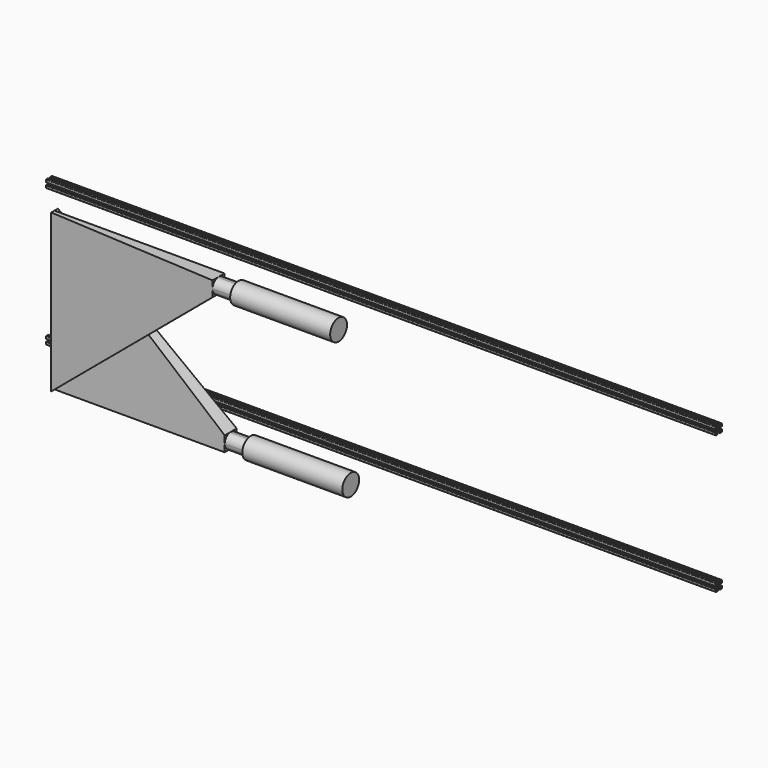
from build123d import *

# Parameters (mm, degrees)
F0_W           = 38.1
F0_H           = 400
F1_DEPTH       = 431.8
F2_SIZE2       = 431.79999
F2_SIZE        = 27.79999
F3_SIZE2       = 27.79999
F3_SIZE        = 431.79999
F4_SIZE2       = 362.19999
F4_SIZE        = 431.79999
F5_SIZE2       = 431.79999
F5_SIZE        = 362.19999
F8_START       = 0.01
F8_DEPTH       = 50.79
F11_START      = 0.01
F9_R           = 26.67
F11_DEPTH      = 253.99
F10_R          = 26.67
F13_DEPTH      = 1600
F13_DEPTH_BACK = 100


# Not quite as in the source:
# - a fillet or chamfer is up to 0.001 mm smaller than in the source, because OpenCascade refuses the exact size
# - ends of sketch curves that miss each other by under 0.0002 mm in the source are joined


with BuildPart() as f1:
    # F0 (on Right) → F1 (new body)
    with BuildSketch(Plane.YZ):
        with Locations((-19.5574148118, 124.7872307897)):
            Rectangle(F0_W, F0_H)
    extrude(amount=F1_DEPTH)

    # F3 (size 431.8 and 27.8 in the source; OpenCascade refuses exactly that, so slightly less here)
    f3_edges = [f1.edges().sort_by_distance(p)[0] for p in [
        (0, -38.607415, 124.787231),
    ]]
    f3_side = f1.faces().sort_by_distance((215.9, -38.607415, 124.787231))[0]
    chamfer(f3_edges, length=F3_SIZE, length2=F3_SIZE2, reference=f3_side)

    # F5 (size 362.2 and 431.8 in the source; OpenCascade refuses exactly that, so slightly less here)
    f5_edges = [f1.edges().sort_by_distance(p)[0] for p in [
        (431.8, -19.557415, -75.212769),
    ]]
    f5_side = f1.faces().sort_by_distance((431.8, -19.557415, 124.787231))[0]
    chamfer(f5_edges, length=F5_SIZE, length2=F5_SIZE2, reference=f5_side)


with BuildPart() as f1b:
    # F0 (on Right) → F1, piece 2 (new body)
    with BuildSketch(Plane.YZ):
        with Locations((19.05, 124.7872307897)):
            Rectangle(F0_W, F0_H)
    extrude(amount=F1_DEPTH)

    # F2 (size 27.8 and 431.8 in the source; OpenCascade refuses exactly that, so slightly less here)
    f2_edges = [f1b.edges().sort_by_distance(p)[0] for p in [
        (0, 38.1, 124.787231),
    ]]
    f2_side = f1b.faces().sort_by_distance((0, 19.05, 124.787231))[0]
    chamfer(f2_edges, length=F2_SIZE, length2=F2_SIZE2, reference=f2_side)

    # F4 (size 431.8 and 362.2 in the source; OpenCascade refuses exactly that, so slightly less here)
    f4_edges = [f1b.edges().sort_by_distance(p)[0] for p in [
        (431.8, 19.05, 324.787231),
    ]]
    f4_side = f1b.faces().sort_by_distance((257.236203, 13.430649, 324.787231))[0]
    chamfer(f4_edges, length=F4_SIZE, length2=F4_SIZE2, reference=f4_side)


with BuildPart() as f8:
    # F6 (on face) → F8 (new body)
    with BuildSketch(Plane.YZ.offset(431.8).offset(F8_START)):
        with BuildLine():
            ThreePointArc((21.4358960581, -75.2127692103), (33.3390486021, -68.911403662), (38.1, -56.3127692103))
            ThreePointArc((38.1, -56.3127692103), (33.3390221993, -43.7141048134), (21.4358168412, -37.4127592103))
            Line((21.4358168412, -37.4127592103), (16.6641831588, -37.4127592103))
            ThreePointArc((16.6641831588, -37.4127592103), (4.7609778007, -43.7141048134), (0, -56.3127692103))
            ThreePointArc((0, -56.3127692103), (4.7609513979, -68.911403662), (16.6641039419, -75.2127692103))
            Line((16.6641039419, -75.2127692103), (21.4358960581, -75.2127692103))
        make_face()
    extrude(amount=F8_DEPTH)


with BuildPart() as f8b:
    # F7 (on face) → F8, piece 2 (new body)
    with BuildSketch(Plane.YZ.offset(431.8).offset(F8_START)):
        with BuildLine():
            ThreePointArc((-17.1715979706, 286.9872207897), (-5.2683926125, 293.2885663927), (-0.5074148118, 305.8872307897))
            ThreePointArc((-0.5074148118, 305.8872307897), (-5.2683662097, 318.4858652413), (-17.1715187538, 324.7872307897))
            Line((-17.1715187538, 324.7872307897), (-21.9433108699, 324.7872307897))
            ThreePointArc((-21.9433108699, 324.7872307897), (-33.846463414, 318.4858652413), (-38.6074148118, 305.8872307897))
            ThreePointArc((-38.6074148118, 305.8872307897), (-33.8464370112, 293.2885663927), (-21.9432316531, 286.9872207897))
            Line((-21.9432316531, 286.9872207897), (-17.1715979706, 286.9872207897))
        make_face()
    extrude(amount=F8_DEPTH)


with BuildPart() as f11:
    # F9 (on face) → F11 (new body)
    with BuildSketch(Plane.YZ.offset(482.6).offset(F11_START)):
        with Locations((-19.5574148118, 305.8872307897)):
            Circle(F9_R)
        with BuildLine():
            ThreePointArc((-17.1715187538, 324.7872307897), (-0.5074148119, 305.8871908669), (-17.1715979706, 286.9872207897))
            Line((-17.1715979706, 286.9872207897), (-21.9432316531, 286.9872207897))
            ThreePointArc((-21.9432316531, 286.9872207897), (-38.6074148118, 305.8871908669), (-21.9433108699, 324.7872307897))
            Line((-21.9433108699, 324.7872307897), (-17.1715187538, 324.7872307897))
        make_face(mode=Mode.SUBTRACT)
        with BuildLine():
            Line((-21.9432316531, 286.9872207897), (-17.1715979706, 286.9872207897))
            ThreePointArc((-17.1715979706, 286.9872207897), (-0.5074148119, 305.8871908669), (-17.1715187538, 324.7872307897))
            Line((-17.1715187538, 324.7872307897), (-21.9433108699, 324.7872307897))
            ThreePointArc((-21.9433108699, 324.7872307897), (-38.6074148118, 305.8871908669), (-21.9432316531, 286.9872207897))
        make_face()
    extrude(amount=F11_DEPTH)


with BuildPart() as f11b:
    # F10 (on face) → F11, piece 2 (new body)
    with BuildSketch(Plane.YZ.offset(482.6).offset(F11_START)):
        with Locations((19.05, -56.3127692103)):
            Circle(F10_R)
        with BuildLine():
            ThreePointArc((21.4358168412, -37.4127592103), (38.1, -56.3127292876), (21.4358960581, -75.2127692103))
            Line((21.4358960581, -75.2127692103), (16.6641039419, -75.2127692103))
            ThreePointArc((16.6641039419, -75.2127692103), (0, -56.3127292876), (16.6641831588, -37.4127592103))
            Line((16.6641831588, -37.4127592103), (21.4358168412, -37.4127592103))
        make_face(mode=Mode.SUBTRACT)
        with BuildLine():
            Line((16.6641039419, -75.2127692103), (21.4358960581, -75.2127692103))
            ThreePointArc((21.4358960581, -75.2127692103), (38.1, -56.3127292876), (21.4358168412, -37.4127592103))
            Line((21.4358168412, -37.4127592103), (16.6641831588, -37.4127592103))
            ThreePointArc((16.6641831588, -37.4127592103), (0, -56.3127292876), (16.6641039419, -75.2127692103))
        make_face()
    extrude(amount=F11_DEPTH)


with BuildPart() as f13:
    # F12 (on Right) → F13 (new body, two sides)
    with BuildSketch(Plane.YZ) as f13_sk:
        with BuildLine():
            Line((84.0865463614, 322.0775318146), (79.3365463614, 322.0775318146))
            ThreePointArc((79.3365463614, 322.0775318146), (78.2758861897, 321.6381919864), (77.8365463614, 320.5775318146))
            Line((77.8365463614, 320.5775318146), (77.8365463614, 315.8275318146))
            ThreePointArc((77.8365463614, 315.8275318146), (77.8951250052, 315.6861104583), (78.0365463614, 315.6275318146))
            Line((78.0365463614, 315.6275318146), (78.1365463614, 315.6275318146))
            ThreePointArc((78.1365463614, 315.6275318146), (78.2779677177, 315.5689531708), (78.3365463614, 315.4275318146))
            Line((78.3365463614, 315.4275318146), (78.3365463614, 315.2775318146))
            ThreePointArc((78.3365463614, 315.2775318146), (78.3951250052, 315.1361104583), (78.5365463614, 315.0775318146))
            Line((78.5365463614, 315.0775318146), (78.8365463614, 315.0775318146))
            ThreePointArc((78.8365463614, 315.0775318146), (79.190099752, 315.223978424), (79.3365463614, 315.5775318146))
            Line((79.3365463614, 315.5775318146), (79.3365463614, 317.5775318146))
            ThreePointArc((79.3365463614, 317.5775318146), (79.4829929709, 317.9310852052), (79.8365463614, 318.0775318146))
            Line((79.8365463614, 318.0775318146), (80.5687763614, 318.0775318146))
            ThreePointArc((80.5687763614, 318.0775318146), (80.760121344, 318.0394702278), (80.922334752, 317.9310802052))
            Line((80.922334752, 317.9310802052), (83.1900963614, 315.6633218146))
            ThreePointArc((83.1900963614, 315.6633218146), (83.2984847747, 315.5011067971), (83.3365463614, 315.3097618146))
            Line((83.3365463614, 315.3097618146), (83.3365463614, 313.0311218146))
            ThreePointArc((83.3365463614, 313.0311218146), (83.3433615249, 312.9793567786), (83.3633425509, 312.9311196145))
            Line((83.3633425509, 312.9311196145), (83.7984263614, 312.1775318146))
            ThreePointArc((83.7984263614, 312.1775318146), (83.8252263614, 312.0775318146), (83.798430172, 311.9775296145))
            Line((83.798430172, 311.9775296145), (83.3633463614, 311.2239418146))
            ThreePointArc((83.3633463614, 311.2239418146), (83.3433615249, 311.1757068505), (83.3365463614, 311.1239418146))
            Line((83.3365463614, 311.1239418146), (83.3365463614, 308.8453018146))
            ThreePointArc((83.3365463614, 308.8453018146), (83.2984847747, 308.653956832), (83.190094752, 308.491743424))
            Line((83.190094752, 308.491743424), (80.9223363614, 306.2239818146))
            ThreePointArc((80.9223363614, 306.2239818146), (80.760121344, 306.1155934013), (80.5687763614, 306.0775318146))
            Line((80.5687763614, 306.0775318146), (79.8365463614, 306.0775318146))
            ThreePointArc((79.8365463614, 306.0775318146), (79.4829929709, 306.223978424), (79.3365463614, 306.5775318146))
            Line((79.3365463614, 306.5775318146), (79.3365463614, 308.5775318146))
            ThreePointArc((79.3365463614, 308.5775318146), (79.190099752, 308.9310852052), (78.8365463614, 309.0775318146))
            Line((78.8365463614, 309.0775318146), (78.5365463614, 309.0775318146))
            ThreePointArc((78.5365463614, 309.0775318146), (78.3951250052, 309.0189531708), (78.3365463614, 308.8775318146))
            Line((78.3365463614, 308.8775318146), (78.3365463614, 308.7275318146))
            ThreePointArc((78.3365463614, 308.7275318146), (78.2779677177, 308.5861104583), (78.1365463614, 308.5275318146))
            Line((78.1365463614, 308.5275318146), (78.0365463614, 308.5275318146))
            ThreePointArc((78.0365463614, 308.5275318146), (77.8951250052, 308.4689531708), (77.8365463614, 308.3275318146))
            Line((77.8365463614, 308.3275318146), (77.8365463614, 303.5775318146))
            ThreePointArc((77.8365463614, 303.5775318146), (78.2758861897, 302.5168716428), (79.3365463614, 302.0775318146))
            Line((79.3365463614, 302.0775318146), (84.0865463614, 302.0775318146))
            ThreePointArc((84.0865463614, 302.0775318146), (84.2279677177, 302.1361104583), (84.2865463614, 302.2775318146))
            Line((84.2865463614, 302.2775318146), (84.2865463614, 302.3775318146))
            ThreePointArc((84.2865463614, 302.3775318146), (84.3451250052, 302.5189531708), (84.4865463614, 302.5775318146))
            Line((84.4865463614, 302.5775318146), (84.6365463614, 302.5775318146))
            ThreePointArc((84.6365463614, 302.5775318146), (84.7779677177, 302.6361104583), (84.8365463614, 302.7775318146))
            Line((84.8365463614, 302.7775318146), (84.8365463614, 303.0775318146))
            ThreePointArc((84.8365463614, 303.0775318146), (84.690099752, 303.4310852052), (84.3365463614, 303.5775318146))
            Line((84.3365463614, 303.5775318146), (82.3365463614, 303.5775318146))
            ThreePointArc((82.3365463614, 303.5775318146), (81.9829929709, 303.723978424), (81.8365463614, 304.0775318146))
            Line((81.8365463614, 304.0775318146), (81.8365463614, 304.8097618146))
            ThreePointArc((81.8365463614, 304.8097618146), (81.8746079482, 305.0011067971), (81.9829979709, 305.1633202051))
            Line((81.9829979709, 305.1633202051), (84.2507563614, 307.4310818146))
            ThreePointArc((84.2507563614, 307.4310818146), (84.4129713789, 307.5394702278), (84.6043163614, 307.5775318146))
            Line((84.6043163614, 307.5775318146), (86.8829563614, 307.5775318146))
            ThreePointArc((86.8829563614, 307.5775318146), (86.9347189826, 307.584346331), (86.9829542314, 307.604325504))
            Line((86.9829542314, 307.604325504), (87.7365463614, 308.0394118146))
            ThreePointArc((87.7365463614, 308.0394118146), (87.8365463614, 308.0662118146), (87.9365485615, 308.0394156251))
            Line((87.9365485615, 308.0394156251), (88.6901363614, 307.6043218146))
            ThreePointArc((88.6901363614, 307.6043218146), (88.7383737403, 307.584346331), (88.7901363614, 307.5775318146))
            Line((88.7901363614, 307.5775318146), (91.0687763614, 307.5775318146))
            ThreePointArc((91.0687763614, 307.5775318146), (91.260121344, 307.5394702278), (91.422334752, 307.4310802052))
            Line((91.422334752, 307.4310802052), (93.6900963614, 305.1633218146))
            ThreePointArc((93.6900963614, 305.1633218146), (93.7984847747, 305.0011067971), (93.8365463614, 304.8097618146))
            Line((93.8365463614, 304.8097618146), (93.8365463614, 304.0775318146))
            ThreePointArc((93.8365463614, 304.0775318146), (93.690099752, 303.723978424), (93.3365463614, 303.5775318146))
            Line((93.3365463614, 303.5775318146), (91.3365463614, 303.5775318146))
            ThreePointArc((91.3365463614, 303.5775318146), (90.9829929709, 303.4310852052), (90.8365463614, 303.0775318146))
            Line((90.8365463614, 303.0775318146), (90.8365463614, 302.7775318146))
            ThreePointArc((90.8365463614, 302.7775318146), (90.8951250052, 302.6361104583), (91.0365463614, 302.5775318146))
            Line((91.0365463614, 302.5775318146), (91.1865463614, 302.5775318146))
            ThreePointArc((91.1865463614, 302.5775318146), (91.3279677177, 302.5189531708), (91.3865463614, 302.3775318146))
            Line((91.3865463614, 302.3775318146), (91.3865463614, 302.2775318146))
            ThreePointArc((91.3865463614, 302.2775318146), (91.4451250052, 302.1361104583), (91.5865463614, 302.0775318146))
            Line((91.5865463614, 302.0775318146), (96.3365463614, 302.0775318146))
            ThreePointArc((96.3365463614, 302.0775318146), (97.3972065332, 302.5168716428), (97.8365463614, 303.5775318146))
            Line((97.8365463614, 303.5775318146), (97.8365463614, 308.3275318146))
            ThreePointArc((97.8365463614, 308.3275318146), (97.7779677177, 308.4689531708), (97.6365463614, 308.5275318146))
            Line((97.6365463614, 308.5275318146), (97.5365463614, 308.5275318146))
            ThreePointArc((97.5365463614, 308.5275318146), (97.3951250052, 308.5861104583), (97.3365463614, 308.7275318146))
            Line((97.3365463614, 308.7275318146), (97.3365463614, 308.8775318146))
            ThreePointArc((97.3365463614, 308.8775318146), (97.2779677177, 309.0189531708), (97.1365463614, 309.0775318146))
            Line((97.1365463614, 309.0775318146), (96.8365463614, 309.0775318146))
            ThreePointArc((96.8365463614, 309.0775318146), (96.4829929709, 308.9310852052), (96.3365463614, 308.5775318146))
            Line((96.3365463614, 308.5775318146), (96.3365463614, 306.5775318146))
            ThreePointArc((96.3365463614, 306.5775318146), (96.190099752, 306.223978424), (95.8365463614, 306.0775318146))
            Line((95.8365463614, 306.0775318146), (95.1043163614, 306.0775318146))
            ThreePointArc((95.1043163614, 306.0775318146), (94.9129713789, 306.1155934013), (94.7507579709, 306.223983424))
            Line((94.7507579709, 306.223983424), (92.4829963614, 308.4917418146))
            ThreePointArc((92.4829963614, 308.4917418146), (92.3746079482, 308.653956832), (92.3365463614, 308.8453018146))
            Line((92.3365463614, 308.8453018146), (92.3365463614, 311.1239418146))
            ThreePointArc((92.3365463614, 311.1239418146), (92.3297311979, 311.1757068505), (92.309750172, 311.2239440146))
            Line((92.309750172, 311.2239440146), (91.8746663614, 311.9775318146))
            ThreePointArc((91.8746663614, 311.9775318146), (91.8478663614, 312.0775318146), (91.8746625509, 312.1775340146))
            Line((91.8746625509, 312.1775340146), (92.3097463614, 312.9311218146))
            ThreePointArc((92.3097463614, 312.9311218146), (92.3297311979, 312.9793567786), (92.3365463614, 313.0311218146))
            Line((92.3365463614, 313.0311218146), (92.3365463614, 315.3097618146))
            ThreePointArc((92.3365463614, 315.3097618146), (92.3746079482, 315.5011067971), (92.4829979709, 315.6633202051))
            Line((92.4829979709, 315.6633202051), (94.7507563614, 317.9310818146))
            ThreePointArc((94.7507563614, 317.9310818146), (94.9129713789, 318.0394702278), (95.1043163614, 318.0775318146))
            Line((95.1043163614, 318.0775318146), (95.8365463614, 318.0775318146))
            ThreePointArc((95.8365463614, 318.0775318146), (96.190099752, 317.9310852052), (96.3365463614, 317.5775318146))
            Line((96.3365463614, 317.5775318146), (96.3365463614, 315.5775318146))
            ThreePointArc((96.3365463614, 315.5775318146), (96.4829929709, 315.223978424), (96.8365463614, 315.0775318146))
            Line((96.8365463614, 315.0775318146), (97.1365463614, 315.0775318146))
            ThreePointArc((97.1365463614, 315.0775318146), (97.2779677177, 315.1361104583), (97.3365463614, 315.2775318146))
            Line((97.3365463614, 315.2775318146), (97.3365463614, 315.4275318146))
            ThreePointArc((97.3365463614, 315.4275318146), (97.3951250052, 315.5689531708), (97.5365463614, 315.6275318146))
            Line((97.5365463614, 315.6275318146), (97.6365463614, 315.6275318146))
            ThreePointArc((97.6365463614, 315.6275318146), (97.7779677177, 315.6861104583), (97.8365463614, 315.8275318146))
            Line((97.8365463614, 315.8275318146), (97.8365463614, 320.5775318146))
            ThreePointArc((97.8365463614, 320.5775318146), (97.3972065332, 321.6381919864), (96.3365463614, 322.0775318146))
            Line((96.3365463614, 322.0775318146), (91.5865463614, 322.0775318146))
            ThreePointArc((91.5865463614, 322.0775318146), (91.4451250052, 322.0189531708), (91.3865463614, 321.8775318146))
            Line((91.3865463614, 321.8775318146), (91.3865463614, 321.7775318146))
            ThreePointArc((91.3865463614, 321.7775318146), (91.3279677177, 321.6361104583), (91.1865463614, 321.5775318146))
            Line((91.1865463614, 321.5775318146), (91.0365463614, 321.5775318146))
            ThreePointArc((91.0365463614, 321.5775318146), (90.8951250052, 321.5189531708), (90.8365463614, 321.3775318146))
            Line((90.8365463614, 321.3775318146), (90.8365463614, 321.0775318146))
            ThreePointArc((90.8365463614, 321.0775318146), (90.9829929709, 320.723978424), (91.3365463614, 320.5775318146))
            Line((91.3365463614, 320.5775318146), (93.3365463614, 320.5775318146))
            ThreePointArc((93.3365463614, 320.5775318146), (93.690099752, 320.4310852052), (93.8365463614, 320.0775318146))
            Line((93.8365463614, 320.0775318146), (93.8365463614, 319.3453018146))
            ThreePointArc((93.8365463614, 319.3453018146), (93.7984847747, 319.153956832), (93.690094752, 318.991743424))
            Line((93.690094752, 318.991743424), (91.4223363614, 316.7239818146))
            ThreePointArc((91.4223363614, 316.7239818146), (91.260121344, 316.6155934013), (91.0687763614, 316.5775318146))
            Line((91.0687763614, 316.5775318146), (88.7901363614, 316.5775318146))
            ThreePointArc((88.7901363614, 316.5775318146), (88.7383737403, 316.5707172981), (88.6901384915, 316.5507381251))
            Line((88.6901384915, 316.5507381251), (87.9365463614, 316.1156518146))
            ThreePointArc((87.9365463614, 316.1156518146), (87.8365463614, 316.0888518146), (87.7365441614, 316.115648004))
            Line((87.7365441614, 316.115648004), (86.9829563614, 316.5507418146))
            ThreePointArc((86.9829563614, 316.5507418146), (86.9347189826, 316.5707172981), (86.8829563614, 316.5775318146))
            Line((86.8829563614, 316.5775318146), (84.6043163614, 316.5775318146))
            ThreePointArc((84.6043163614, 316.5775318146), (84.4129713789, 316.6155934013), (84.2507579709, 316.723983424))
            Line((84.2507579709, 316.723983424), (81.9829963614, 318.9917418146))
            ThreePointArc((81.9829963614, 318.9917418146), (81.8746079482, 319.153956832), (81.8365463614, 319.3453018146))
            Line((81.8365463614, 319.3453018146), (81.8365463614, 320.0775318146))
            ThreePointArc((81.8365463614, 320.0775318146), (81.9829929709, 320.4310852052), (82.3365463614, 320.5775318146))
            Line((82.3365463614, 320.5775318146), (84.3365463614, 320.5775318146))
            ThreePointArc((84.3365463614, 320.5775318146), (84.690099752, 320.723978424), (84.8365463614, 321.0775318146))
            Line((84.8365463614, 321.0775318146), (84.8365463614, 321.3775318146))
            ThreePointArc((84.8365463614, 321.3775318146), (84.7779677177, 321.5189531708), (84.6365463614, 321.5775318146))
            Line((84.6365463614, 321.5775318146), (84.4865463614, 321.5775318146))
            ThreePointArc((84.4865463614, 321.5775318146), (84.3451250052, 321.6361104583), (84.2865463614, 321.7775318146))
            Line((84.2865463614, 321.7775318146), (84.2865463614, 321.8775318146))
            ThreePointArc((84.2865463614, 321.8775318146), (84.2279677177, 322.0189531708), (84.0865463614, 322.0775318146))
        make_face()
        with BuildLine():
            ThreePointArc((84.844373496, 313.9874636436), (85.3248090058, 314.5859403747), (85.9226480695, 315.0671691465))
            Line((85.9226480695, 315.0671691465), (86.5783563614, 314.5228318146))
            ThreePointArc((86.5783563614, 314.5228318146), (87.8365463614, 314.8275318146), (89.0947335193, 314.5228262909))
            Line((89.0947335193, 314.5228262909), (89.7504463614, 315.0671718146))
            ThreePointArc((89.7504463614, 315.0671718146), (90.3482837171, 314.5859403747), (90.8287192269, 313.9874636436))
            Line((90.8287192269, 313.9874636436), (90.2818463614, 313.3357218146))
            ThreePointArc((90.2818463614, 313.3357218146), (90.5865463614, 312.0775318146), (90.2818408377, 310.8193446567))
            Line((90.2818408377, 310.8193446567), (90.8287163614, 310.1676018146))
            ThreePointArc((90.8287163614, 310.1676018146), (90.3482837171, 309.5691232544), (89.7504446534, 309.0878944827))
            Line((89.7504446534, 309.0878944827), (89.0947363614, 309.6322318146))
            ThreePointArc((89.0947363614, 309.6322318146), (87.8365463614, 309.3275318146), (86.5783592036, 309.6322373383))
            Line((86.5783592036, 309.6322373383), (85.9226463614, 309.0878918146))
            ThreePointArc((85.9226463614, 309.0878918146), (85.3248090058, 309.5691232544), (84.844373496, 310.1675999855))
            Line((84.844373496, 310.1675999855), (85.3912463614, 310.8193418146))
            ThreePointArc((85.3912463614, 310.8193418146), (85.0865463614, 312.0775318146), (85.3912518852, 313.3357189724))
            Line((85.3912518852, 313.3357189724), (84.844373496, 313.9874636436))
        make_face(mode=Mode.SUBTRACT)
    extrude(amount=F13_DEPTH)
    extrude(f13_sk.sketch, amount=-F13_DEPTH_BACK)


with BuildPart() as f14_1:
    # F14: copy of F13
    add(f13.part.moved(Location((0, 0, -350))))


with BuildPart() as f14_1_1:
    # F15: moved
    add(f14_1.part.moved(Location((0, 20, 0))))


with BuildPart() as f13_1:
    # F15: moved
    add(f13.part.moved(Location((0, 20, 0))))


solid = Compound([f1.part, f1b.part, f8.part, f8b.part, f11.part, f11b.part, f14_1_1.part, f13_1.part])
